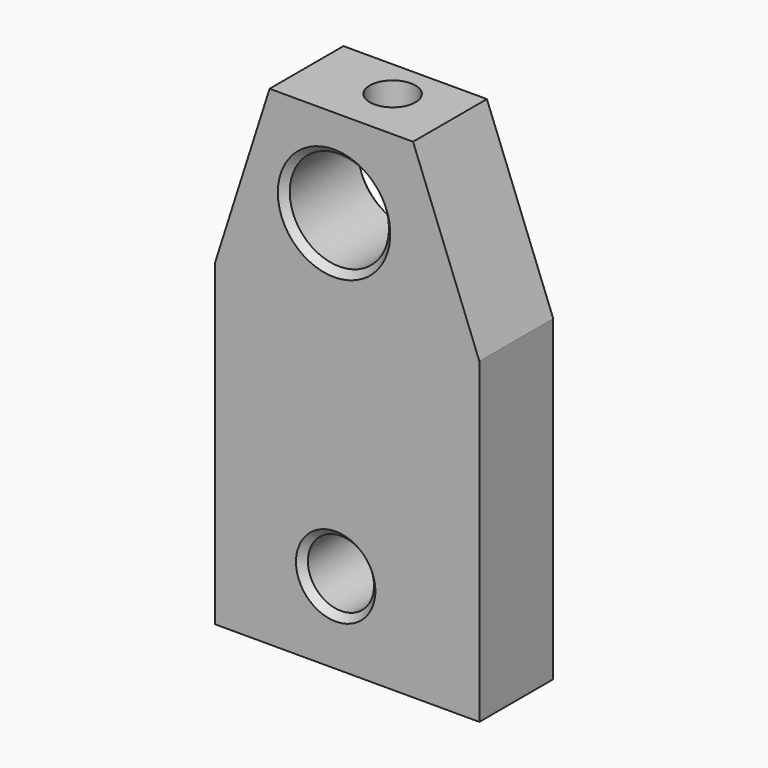
from build123d import *

# Parameters (mm, degrees)
F1_DEPTH = 18.9992
F3_D     = 19.05
F4_D     = 12.7
F5_R     = 4.3873111452
F6_DEPTH = 25.4
F7_SIZE  = 1.27


with BuildPart() as f1:
    # F0 (on Front) → F1 (new body)
    with BuildSketch(Plane.XZ):
        Polygon((-52.6177957654, 0), (-52.6177957654, -60.96), (-1.8177957654, -60.96), (-1.8177957654, 0), (-14.5472735167, 32.9634994268), (-34.6658416092, 32.9634994268), (-42.0942343771, 32.9634994268), align=None)
    extrude(amount=F1_DEPTH)

    # F3 (through all)
    with Locations(Plane.XZ.offset(18.9992)):
        with Locations((-29.7135785222, 15.9400962293)):
            Hole(F3_D / 2)

    # F4 (through all)
    with Locations(Plane.XZ.offset(18.9992)):
        with Locations((-29.4040627778, -45.3441590071)):
            Hole(F4_D / 2)

    # F5 (on face) → F6 (cut)
    with BuildSketch(Plane.XY.offset(32.9634994268)):
        with Locations((-26.6399271786, -8.7757343426)):
            Circle(F5_R)
    extrude(amount=-F6_DEPTH, mode=Mode.SUBTRACT)

    # F7
    f7_edges = [f1.edges().sort_by_distance(p)[0] for p in [
        (-47.356015, 0, 16.48175),
        (-52.617796, 0, -30.48),
        (-1.817796, 0, -30.48),
        (-8.182535, 0, 16.48175),
        (-28.320754, 0, 32.963499),
        (-35.754063, -18.9992, -45.344159),
        (-39.238579, -18.9992, 15.940096),
        (-39.238579, 0, 15.940096),
        (-35.754063, 0, -45.344159),
    ]]
    chamfer(f7_edges, length=F7_SIZE)


solid = f1.part
